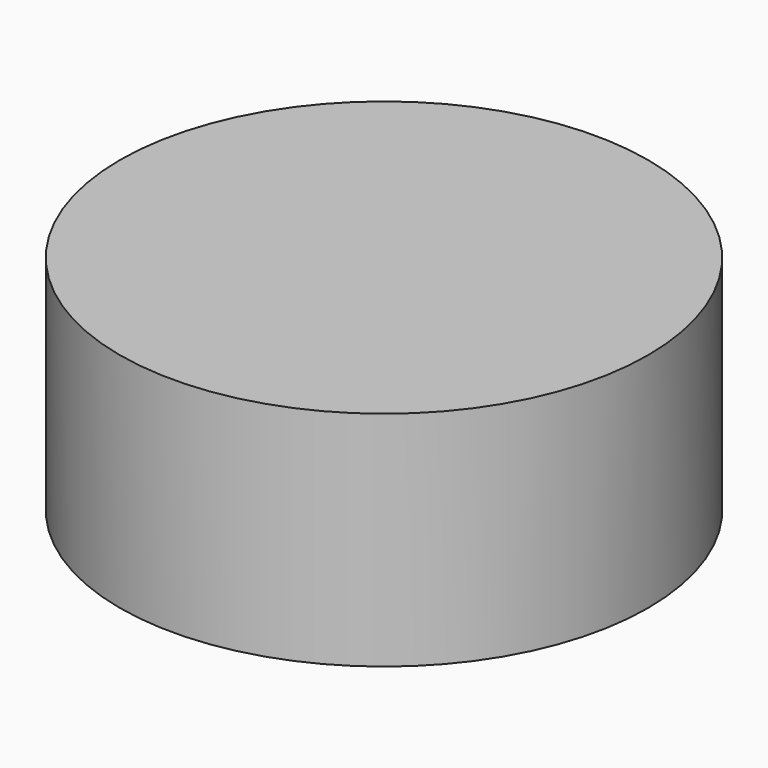
from build123d import *

# Parameters (mm, degrees)
F0_R     = 30.1369846968
F1_DEPTH = 25.4


# Not quite as in the source:
# - the program builds the solid bodies; features that only make, move or delete a surface that nothing else refers to are left out


with BuildPart() as f1:
    # F0 (on Top) → F1 (new body)
    with BuildSketch(Plane.XY):
        with Locations((-46.9826161861, 26.7940461636)):
            Circle(F0_R)
    extrude(amount=F1_DEPTH)


solid = f1.part
